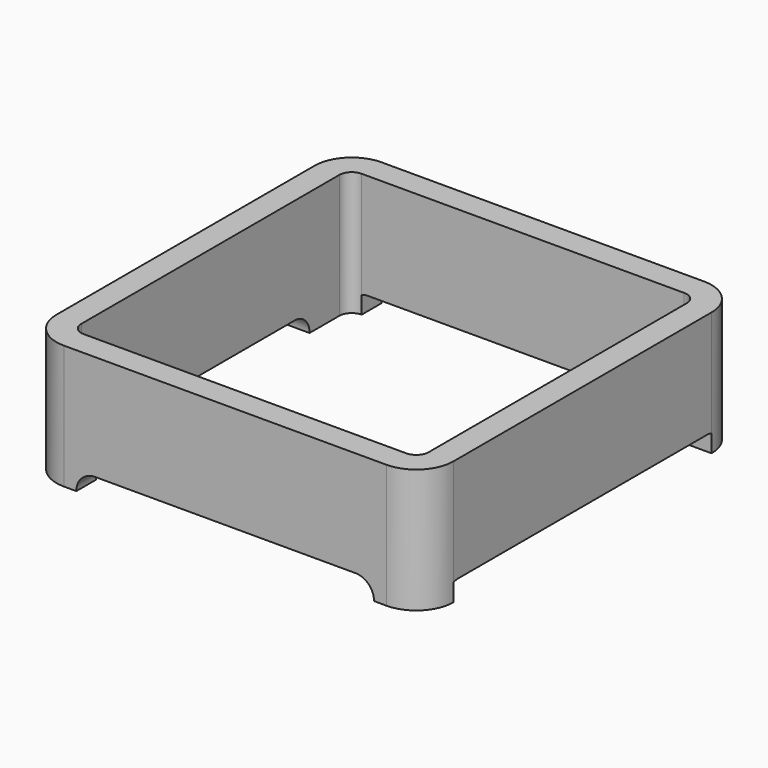
from build123d import *

# Parameters (mm, degrees)
F0_W      = 101.6
F0_H      = 101.6
F1_DEPTH  = 31.75
F2_R      = 9.525
F3_T      = -6.35
F8_DEPTH  = 6.35
F9_DEPTH  = 6.35
F10_DEPTH = 6.35
F11_DEPTH = 6.35


# Not quite as in the source:
# - a feature names something its author has since deleted; it is built from what else it names


with BuildPart() as f1:
    # F0 (on Top) → F1 (new body)
    with BuildSketch(Plane.XY):
        with Locations((50.8, -50.8)):
            Rectangle(F0_W, F0_H)
    extrude(amount=F1_DEPTH)

    # F2
    f2_edges = [f1.edges().sort_by_distance(p)[0] for p in [
        (0, -101.6, 15.875),
        (0, 0, 15.875),
        (101.6, 0, 15.875),
        (101.6, -101.6, 15.875),
    ]]
    fillet(f2_edges, radius=F2_R)

    # F3
    f3_openings = [f1.faces().sort_by_distance(p)[0] for p in [
        (50.8, -50.8, 0),
        (50.8, -50.8, 31.75),
    ]]
    offset(amount=F3_T, openings=f3_openings)

    # F6 (on face) → F8 (cut, through all)
    with BuildSketch(Plane(origin=(0, 0, 0), x_dir=(-1, 0, 0), z_dir=(0, 1, 0))):
        with BuildLine():
            Line((-50.8, 4.7625), (-90.4875, 4.7625))
            ThreePointArc((-90.4875, 4.7625), (-91.2928481737, 4.6939131403), (-92.075, 4.4901280605))
            Line((-92.075, 4.4901280605), (-92.075, 0))
            Line((-92.075, 0), (-9.525, 0))
            Line((-9.525, 0), (-9.525, 4.4901280605))
            ThreePointArc((-9.525, 4.4901280605), (-10.3071518263, 4.6939131403), (-11.1125, 4.7625))
            Line((-11.1125, 4.7625), (-50.8, 4.7625))
        make_face()
    extrude(amount=-F8_DEPTH, mode=Mode.SUBTRACT)

    # F7 (on face) → F9 (cut, through all)
    with BuildSketch(Plane.YZ.offset(101.6)):
        with BuildLine():
            Line((-50.8, 4.7625), (-90.4875, 4.7625))
            ThreePointArc((-90.4875, 4.7625), (-91.2928481737, 4.6939131403), (-92.075, 4.4901280605))
            Line((-92.075, 4.4901280605), (-92.075, 0))
            Line((-92.075, 0), (-9.525, 0))
            Line((-9.525, 0), (-9.525, 4.4901280605))
            ThreePointArc((-9.525, 4.4901280605), (-10.3071518263, 4.6939131403), (-11.1125, 4.7625))
            Line((-11.1125, 4.7625), (-50.8, 4.7625))
        make_face()
    extrude(amount=-F9_DEPTH, mode=Mode.SUBTRACT)

    # F4 (on face) → F10 (cut, through all)
    with BuildSketch(Plane.XZ.offset(101.6)):
        with BuildLine():
            Line((50.8, 4.7625), (17.4625, 4.7625))
            ThreePointArc((17.4625, 4.7625), (14.0949039546, 3.3675960454), (12.7, 0))
            Line((12.7, 0), (88.9, 0))
            ThreePointArc((88.9, 0), (87.5050960454, 3.3675960454), (84.1375, 4.7625))
            Line((84.1375, 4.7625), (50.8, 4.7625))
        make_face()
    extrude(amount=-F10_DEPTH, mode=Mode.SUBTRACT)

    # F5 (on face) → F11 (cut, through all)
    with BuildSketch(Plane(origin=(0, 0, 0), x_dir=(0, -1, 0), z_dir=(-1, 0, 0))):
        with BuildLine():
            Line((50.8, 4.7625), (23.8125, 4.7625))
            ThreePointArc((23.8125, 4.7625), (20.4449039546, 3.3675960454), (19.05, 0))
            Line((19.05, 0), (82.55, 0))
            ThreePointArc((82.55, 0), (81.1550960454, 3.3675960454), (77.7875, 4.7625))
            Line((77.7875, 4.7625), (50.8, 4.7625))
        make_face()
    extrude(amount=-F11_DEPTH, mode=Mode.SUBTRACT)


solid = f1.part
